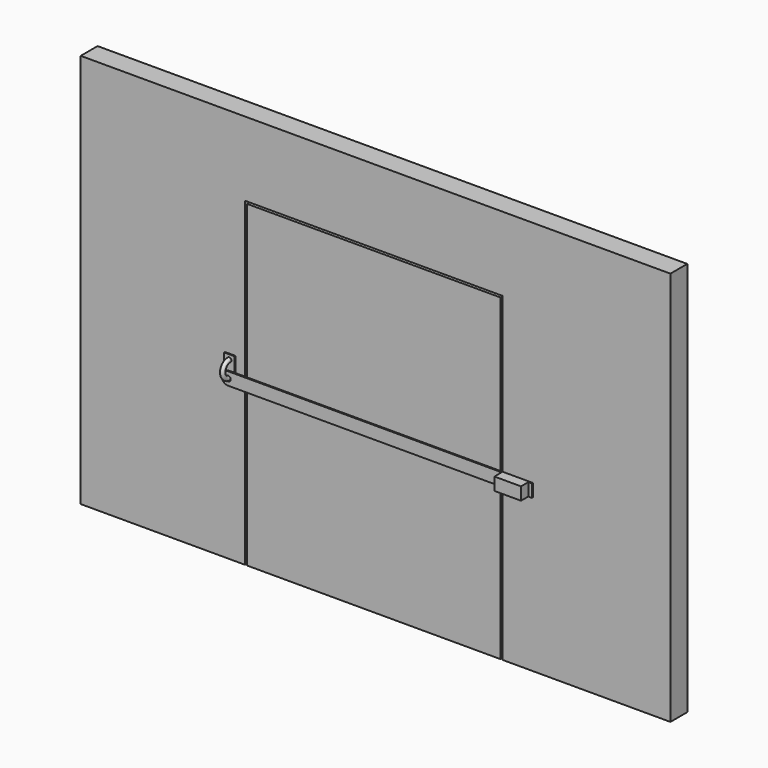
from build123d import *

# Parameters (mm, degrees)
F1_W      = 1200
F1_H      = 1508.9189000277
F2_DEPTH  = 100
F4_R      = 12.5
F5_DEPTH  = 6
F9_R      = 10
F11_W     = 50
F11_H     = 120
F12_DEPTH = 5
F13_R     = 17.5
F13_R_2   = 10.25
F14_DEPTH = 2
F16_DEPTH = 12
F18_DEPTH = 138.001
F22_R     = 6
F24_R     = 10
F24_R_2   = 6
F25_DEPTH = 2
F27_DEPTH = 12
F29_DEPTH = 40
F30_W     = 126
F30_H     = 60
F31_DEPTH = 3


with BuildPart() as f2:
    # F1 (on Front) → F2 (new body)
    with BuildSketch(Plane.XZ):
        with Locations((-16.2692907102, -136.2927497408)):
            Rectangle(F1_W, F1_H)
    extrude(amount=-F2_DEPTH)


with BuildPart() as f2b:
    # F1 (on Front) → F2, piece 2 (new body)
    with BuildSketch(Plane.XZ):
        Polygon((-626.2692907102, 979.5180817103), (-1404.6476536957, 979.5180817103), (-1404.6476536957, -890.7521997547), (-626.2692907102, -890.7521997547), (-626.2692907102, 628.166700273), (593.7307092898, 628.166700273), (593.7307092898, -890.7521997547), (1389.9468982188, -890.7521997547), (1389.9468982188, 979.5180817103), (593.7307092898, 979.5180817103), align=None)
    extrude(amount=-F2_DEPTH)


with BuildPart() as f5:
    # F4 (on offset) → F5 (new body)
    with BuildSketch(Plane.XZ.offset(7)):
        with BuildLine():
            Line((743.7307092898, -100.8483727276), (-696.2692907102, -100.8483727276))
            ThreePointArc((-696.2692907102, -100.8483727276), (-717.4824941458, -109.635169292), (-726.2692907102, -130.8483727276))
            ThreePointArc((-726.2692907102, -130.8483727276), (-717.4824941458, -152.0615761632), (-696.2692907102, -160.8483727276))
            Line((-696.2692907102, -160.8483727276), (743.7307092898, -160.8483727276))
            Line((743.7307092898, -160.8483727276), (743.7307092898, -100.8483727276))
        make_face()
        with Locations((-696.2692907102, -130.8483727276)):
            Circle(F4_R, mode=Mode.SUBTRACT)
    extrude(amount=F5_DEPTH)

    # F17 (on face) → F18 (cut, through all)
    with BuildSketch(Plane.XZ.offset(13)):
        with BuildLine():
            Line((686.7307092898, -123.8483727276), (640.7307092898, -123.8483727276))
            ThreePointArc((640.7307092898, -123.8483727276), (635.7809618215, -125.8986252593), (633.7307092898, -130.8483727276))
            ThreePointArc((633.7307092898, -130.8483727276), (635.7809618215, -135.7981201959), (640.7307092898, -137.8483727276))
            Line((640.7307092898, -137.8483727276), (686.7307092898, -137.8483727276))
            ThreePointArc((686.7307092898, -137.8483727276), (691.6804567581, -135.7981201959), (693.7307092898, -130.8483727276))
            ThreePointArc((693.7307092898, -130.8483727276), (691.6804567581, -125.8986252593), (686.7307092898, -123.8483727276))
        make_face()
    extrude(amount=-F18_DEPTH, mode=Mode.SUBTRACT)

    # F28 (on face) → F29 (join)
    with BuildSketch(Plane.XZ.offset(13)):
        Polygon((600.7307092898, -160.8483727276), (603.7307092898, -160.8483727276), (603.7307092898, -103.8483727276), (723.7307092898, -103.8483727276), (723.7307092898, -160.8483727276), (726.7307092898, -160.8483727276), (726.7307092898, -100.8483727276), (600.7307092898, -100.8483727276), align=None)
    extrude(amount=F29_DEPTH)

    # F30 (on face) → F31 (join)
    with BuildSketch(Plane.XZ.offset(53)):
        with Locations((663.7307092898, -130.8483727276)):
            Rectangle(F30_W, F30_H)
    extrude(amount=F31_DEPTH)


with BuildPart() as f10:
    # F10: sweep along a path in F7
    with BuildLine(Plane(origin=(-696.2692907102, 0, 0), x_dir=(0, -1, 0), z_dir=(-1, 0, 0))) as f10_path:
        Line((-125, -55.8483727276), (7, -55.8483727276))
        ThreePointArc((7, -55.8483727276), (44.5, -93.3483727276), (7, -130.8483727276))
        Line((7, -130.8483727276), (-125, -130.8483727276))
    # F9 (on line) → F10 (sweep)
    with BuildSketch(Plane(origin=(0, 125, 0), x_dir=(-1, 0, 0), z_dir=(0, 1, 0))):
        with Locations((696.2692907102, -55.8483727276)):
            Circle(F9_R)
    sweep(path=f10_path.line)

    # F11 (on face) → F12 (join)
    with BuildSketch(Plane.XZ):
        with Locations((-696.2692907102, -93.7452787161)):
            Rectangle(F11_W, F11_H)
    extrude(amount=F12_DEPTH)


with BuildPart() as f14:
    # F13 (on face) → F14 (new body)
    with BuildSketch(Plane(origin=(0, 100, 0), x_dir=(-1, 0, 0), z_dir=(0, 1, 0))):
        with Locations((696.2692907102, -55.8483727276)):
            Circle(F13_R)
        with Locations((696.2692907102, -55.8483727276)):
            Circle(F13_R_2, mode=Mode.SUBTRACT)
    extrude(amount=F14_DEPTH)


with BuildPart() as f14b:
    # F13 (on face) → F14, piece 2 (new body)
    with BuildSketch(Plane(origin=(0, 100, 0), x_dir=(-1, 0, 0), z_dir=(0, 1, 0))):
        with Locations((696.2692907102, -130.8483727276)):
            Circle(F13_R)
        with Locations((696.2692907102, -130.8483727276)):
            Circle(F13_R_2, mode=Mode.SUBTRACT)
    extrude(amount=F14_DEPTH)


with BuildPart() as f16:
    # F15 (on face) → F16 (new body)
    with BuildSketch(Plane(origin=(0, 102, 0), x_dir=(-1, 0, 0), z_dir=(0, 1, 0))):
        Polygon((700.2425423067, -69.122907437), (709.7520007902, -59.0447032641), (705.7787491936, -45.7701685547), (692.2960391136, -42.5738380183), (682.7865806302, -52.6520421912), (686.7598322267, -65.9265769006), align=None)
    extrude(amount=F16_DEPTH)


with BuildPart() as f16b:
    # F15 (on face) → F16, piece 2 (new body)
    with BuildSketch(Plane(origin=(0, 102, 0), x_dir=(-1, 0, 0), z_dir=(0, 1, 0))):
        Polygon((700.2425423067, -144.122907437), (709.7520007902, -134.0447032641), (705.7787491936, -120.7701685547), (692.2960391136, -117.5738380183), (682.7865806302, -127.6520421912), (686.7598322267, -140.9265769006), align=None)
    extrude(amount=F16_DEPTH)


with BuildPart() as f23:
    # F23: sweep along a path in F20
    with BuildLine(Plane.XY.offset(-130.8483727276)) as f23_path:
        Line((643.7307092898, 125), (643.7307092898, -10))
        ThreePointArc((643.7307092898, -10), (663.7307092898, -30), (683.7307092898, -10))
        Line((683.7307092898, -10), (683.7307092898, 125))
    # F22 (on line) → F23 (sweep)
    with BuildSketch(Plane(origin=(0, 125, 0), x_dir=(-1, 0, 0), z_dir=(0, 1, 0))):
        with Locations((-643.7307092898, -130.8483727276)):
            Circle(F22_R)
    sweep(path=f23_path.line)


with BuildPart() as f25:
    # F24 (on face) → F25 (new body)
    with BuildSketch(Plane(origin=(0, 100, 0), x_dir=(-1, 0, 0), z_dir=(0, 1, 0))):
        with Locations((-643.7307092898, -130.8483727276)):
            Circle(F24_R)
        with Locations((-643.7307092898, -130.8483727276)):
            Circle(F24_R_2, mode=Mode.SUBTRACT)
    extrude(amount=F25_DEPTH)


with BuildPart() as f25b:
    # F24 (on face) → F25, piece 2 (new body)
    with BuildSketch(Plane(origin=(0, 100, 0), x_dir=(-1, 0, 0), z_dir=(0, 1, 0))):
        with Locations((-683.7307092898, -130.8483727276)):
            Circle(F24_R)
        with Locations((-683.7307092898, -130.8483727276)):
            Circle(F24_R_2, mode=Mode.SUBTRACT)
    extrude(amount=F25_DEPTH)


with BuildPart() as f27:
    # F26 (on face) → F27 (new body)
    with BuildSketch(Plane(origin=(0, 102, 0), x_dir=(-1, 0, 0), z_dir=(0, 1, 0))):
        Polygon((-645.915261656, -120.0984395049), (-654.1327007328, -127.3652839613), (-651.9481483666, -138.115217184), (-641.5461569237, -141.5983059503), (-633.3287178469, -134.331461494), (-635.5132702131, -123.5815282713), align=None)
    extrude(amount=F27_DEPTH)


with BuildPart() as f27b:
    # F26 (on face) → F27, piece 2 (new body)
    with BuildSketch(Plane(origin=(0, 102, 0), x_dir=(-1, 0, 0), z_dir=(0, 1, 0))):
        Polygon((-684.4996026959, -119.9056977227), (-693.5917905325, -126.0429164476), (-692.8228971264, -136.9855914525), (-682.9618158838, -141.7910477326), (-673.8696280472, -135.6538290076), (-674.6385214532, -124.7111540027), align=None)
    extrude(amount=F27_DEPTH)


solid = Compound([f2.part, f2b.part, f5.part, f10.part, f14.part, f14b.part, f16.part, f16b.part, f23.part, f25.part, f25b.part, f27.part, f27b.part])
